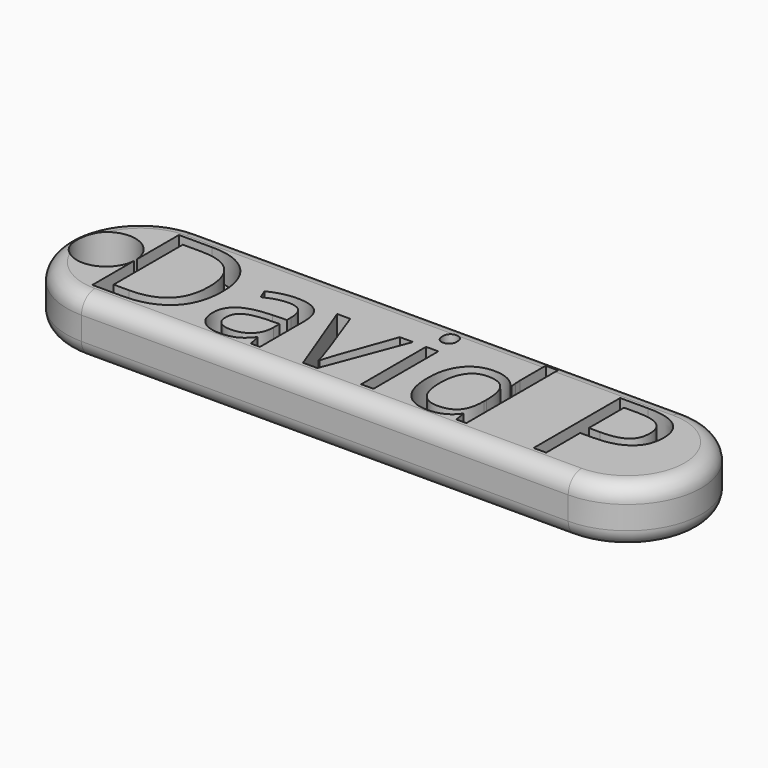
from build123d import *

# Parameters (mm, degrees)
F0_R         = 5.2657436615
F1_DEPTH     = 5.08
F2_TEXT_SIZE = 27.2435485385
F3_DEPTH     = 5.08
F4_T1_DEPTH  = 87.4948054552
F4_T4_ANGLE  = 180
F4_T6_ANGLE  = 180
F4_T8_ANGLE  = 180
F4_T10_ANGLE = 180


# Not quite as in the source:
# - a fillet or chamfer that OpenCascade refuses, or shapes differently, is made with other operations: its cross-section is extruded or revolved along the edge and cut away or added
# - Text() gives the source's letters only with a copy of the font that has no kerning and outlines rounded to 1/6400 em; it was checked with that copy


with BuildPart() as f1:
    # F0 (on Top) → F1 (new body, symmetric)
    with BuildSketch(Plane.XY):
        with BuildLine():
            Line((0, 13.2919847965), (-43.7474027276, 13.2919847965))
            ThreePointArc((-43.7474027276, 13.2919847965), (-57.0393875241, 0), (-43.7474027276, -13.2919847965))
            Line((-43.7474027276, -13.2919847965), (0, -13.2919847965))
            Line((0, -13.2919847965), (43.7474027276, -13.2919847965))
            ThreePointArc((43.7474027276, -13.2919847965), (57.0393875241, 0), (43.7474027276, 13.2919847965))
            Line((43.7474027276, 13.2919847965), (0, 13.2919847965))
        make_face()
        with Locations((-49.9417260289, 0)):
            Circle(F0_R, mode=Mode.SUBTRACT)
    extrude(amount=F1_DEPTH, both=True)

    # F2 (on Top) → F3 (cut)
    with BuildSketch(Plane.XY):
        with Locations((-47.3607592285, -9.6786294598)):
            Text('David P', F2_TEXT_SIZE, font='Open Sans', text_align=(TextAlign.LEFT, TextAlign.BOTTOM))
    extrude(amount=F3_DEPTH, mode=Mode.SUBTRACT)

    # F4: fillet of radius 3 on 2 edges, made by hand

    # F4_s2 → F4_t1 (cut)
    with BuildSketch(Plane.YZ.offset(-43.7474027276)):
        with BuildLine():
            ThreePointArc((13.2919847965, -2.08), (12.4133051401, -4.2013203436), (10.2919847965, -5.08))
            Line((10.2919847965, -5.08), (10.2919847965, -5.14))
            Line((10.2919847965, -5.14), (13.3519847965, -5.14))
            Line((13.3519847965, -5.14), (13.3519847965, -2.08))
            Line((13.3519847965, -2.08), (13.2919847965, -2.08))
        make_face()
        with BuildLine():
            ThreePointArc((-10.2919847965, -5.08), (-12.4133051401, -4.2013203436), (-13.2919847965, -2.08))
            Line((-13.2919847965, -2.08), (-13.3519847965, -2.08))
            Line((-13.3519847965, -2.08), (-13.3519847965, -5.14))
            Line((-13.3519847965, -5.14), (-10.2919847965, -5.14))
            Line((-10.2919847965, -5.14), (-10.2919847965, -5.08))
        make_face()
        with BuildLine():
            ThreePointArc((13.2919847965, 2.08), (12.4133051401, 4.2013203436), (10.2919847965, 5.08))
            Line((10.2919847965, 5.08), (10.2919847965, 5.14))
            Line((10.2919847965, 5.14), (13.3519847965, 5.14))
            Line((13.3519847965, 5.14), (13.3519847965, 2.08))
            Line((13.3519847965, 2.08), (13.2919847965, 2.08))
        make_face()
        with BuildLine():
            ThreePointArc((-10.2919847965, 5.08), (-12.4133051401, 4.2013203436), (-13.2919847965, 2.08))
            Line((-13.2919847965, 2.08), (-13.3519847965, 2.08))
            Line((-13.3519847965, 2.08), (-13.3519847965, 5.14))
            Line((-13.3519847965, 5.14), (-10.2919847965, 5.14))
            Line((-10.2919847965, 5.14), (-10.2919847965, 5.08))
        make_face()
    extrude(amount=F4_T1_DEPTH, mode=Mode.SUBTRACT)

    # F4_s3 → F4_t4 (revolve, cut)
    with BuildSketch(Plane.YZ.offset(-43.7474027276)):
        with BuildLine():
            ThreePointArc((13.2919847965, 2.08), (12.4133051401, 4.2013203436), (10.2919847965, 5.08))
            Line((10.2919847965, 5.08), (10.2919847965, 5.14))
            Line((10.2919847965, 5.14), (13.3519847965, 5.14))
            Line((13.3519847965, 5.14), (13.3519847965, 2.08))
            Line((13.3519847965, 2.08), (13.2919847965, 2.08))
        make_face()
    revolve(axis=Axis((-43.7474027276, 0, 5.08), (0, 0, 1)), revolution_arc=F4_T4_ANGLE, mode=Mode.SUBTRACT)

    # F4_s5 → F4_t6 (revolve, cut)
    with BuildSketch(Plane.YZ.offset(-43.7474027276)):
        with BuildLine():
            ThreePointArc((10.2919847965, -5.08), (12.4133051401, -4.2013203436), (13.2919847965, -2.08))
            Line((13.2919847965, -2.08), (13.3519847965, -2.08))
            Line((13.3519847965, -2.08), (13.3519847965, -5.14))
            Line((13.3519847965, -5.14), (10.2919847965, -5.14))
            Line((10.2919847965, -5.14), (10.2919847965, -5.08))
        make_face()
    revolve(axis=Axis((-43.7474027276, 0, -5.08), (0, 0, 1)), revolution_arc=F4_T6_ANGLE, mode=Mode.SUBTRACT)

    # F4_s7 → F4_t8 (revolve, cut)
    with BuildSketch(Plane.YZ.offset(43.7474027276)):
        with BuildLine():
            ThreePointArc((-10.2919847965, -5.08), (-12.4133051401, -4.2013203436), (-13.2919847965, -2.08))
            Line((-13.2919847965, -2.08), (-13.3519847965, -2.08))
            Line((-13.3519847965, -2.08), (-13.3519847965, -5.14))
            Line((-13.3519847965, -5.14), (-10.2919847965, -5.14))
            Line((-10.2919847965, -5.14), (-10.2919847965, -5.08))
        make_face()
    revolve(axis=Axis((43.7474027276, 0, -5.08), (0, 0, 1)), revolution_arc=F4_T8_ANGLE, mode=Mode.SUBTRACT)

    # F4_s9 → F4_t10 (revolve, cut)
    with BuildSketch(Plane.YZ.offset(43.7474027276)):
        with BuildLine():
            ThreePointArc((-10.2919847965, 5.08), (-12.4133051401, 4.2013203436), (-13.2919847965, 2.08))
            Line((-13.2919847965, 2.08), (-13.3519847965, 2.08))
            Line((-13.3519847965, 2.08), (-13.3519847965, 5.14))
            Line((-13.3519847965, 5.14), (-10.2919847965, 5.14))
            Line((-10.2919847965, 5.14), (-10.2919847965, 5.08))
        make_face()
    revolve(axis=Axis((43.7474027276, 0, 5.08), (0, 0, 1)), revolution_arc=F4_T10_ANGLE, mode=Mode.SUBTRACT)


solid = f1.part
